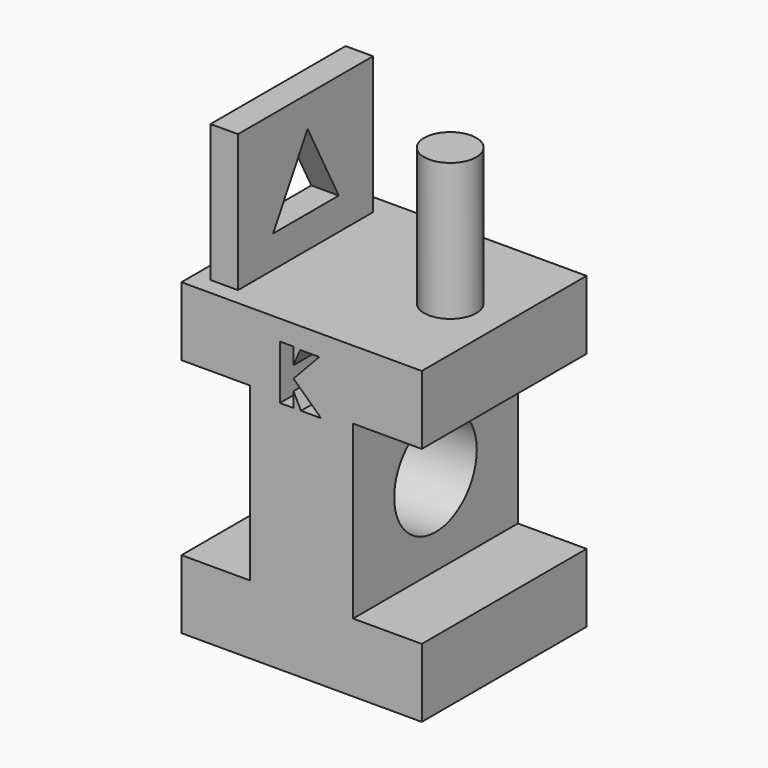
from build123d import *

# Parameters (mm, degrees)
F1_DEPTH  = 76.2
F2_R      = 19.096035609
F3_DEPTH  = 47.498
F4_W      = 10.16
F4_H      = 62.4394440092
F5_DEPTH  = 50.8
F7_DEPTH  = 25.4
F9_DEPTH  = 96.52
F10_R     = 9.6573764136
F11_DEPTH = 50.8


# Not quite as in the source:
# - a feature names something its author has since deleted; it is built from what else it names


with BuildPart() as f1:
    # F0 (on Front) → F1 (new body)
    with BuildSketch(Plane.XZ):
        Polygon((-43.9144560635, -19.0287967878), (-43.9144560635, -44.4287967878), (44.9855439365, -44.4287967878), (44.9855439365, -19.0287967878), (19.5855439365, -19.0287967878), (19.5855439365, 44.4712032122), (44.9855439365, 44.4712032122), (44.9855439365, 69.8712032122), (-43.9144560635, 69.8712032122), (-43.9144560635, 44.4712032122), (-18.5144560635, 44.4712032122), (-18.5144560635, -19.0287967878), align=None)
    extrude(amount=F1_DEPTH)

    # F2 (on face) → F3 (cut)
    with BuildSketch(Plane.YZ.offset(19.5855439365)):
        with Locations((-38.1, 12.7212032122)):
            Circle(F2_R)
    extrude(amount=-F3_DEPTH, mode=Mode.SUBTRACT)

    # F4 (on face) → F5 (join)
    with BuildSketch(Plane.XY.offset(69.8712032122)):
        with Locations((-33.1311938035, -38.6642131489)):
            Rectangle(F4_W, F4_H)
    extrude(amount=F5_DEPTH)

    # F6 (on face) → F7 (cut)
    with BuildSketch(Plane(origin=(-38.2111938035, 0, 0), x_dir=(0, -1, 0), z_dir=(-1, 0, 0))):
        Polygon((53.6283701658, 81.7187428474), (37.7003215253, 109.3182116747), (23.2826862484, 81.7187428474), align=None)
    extrude(amount=-F7_DEPTH, mode=Mode.SUBTRACT)

    # F8 (on face) → F9 (cut)
    with BuildSketch(Plane(origin=(0, 0, 0), x_dir=(-1, 0, 0), z_dir=(0, 1, 0))):
        Polygon((7.511020638, 42.3752516508), (7.511020638, 62.378142029), (2.4668793194, 62.378142029), (2.4668793194, 56.307456918), (0, 62.0944574475), (-7.0838662127, 62.0944574475), (2.4668793194, 51.9569911986), (-7.7034849674, 42.3752516508), (-0.3085337383, 42.3752516508), (2.4668793194, 47.8559471667), (2.4668793194, 42.3752516508), align=None)
    extrude(amount=-F9_DEPTH, mode=Mode.SUBTRACT)

    # F10 (on face) → F11 (join)
    with BuildSketch(Plane.XY.offset(69.8712032122)):
        with Locations((25.0358451158, -38.1)):
            Circle(F10_R)
    extrude(amount=F11_DEPTH)


solid = f1.part
